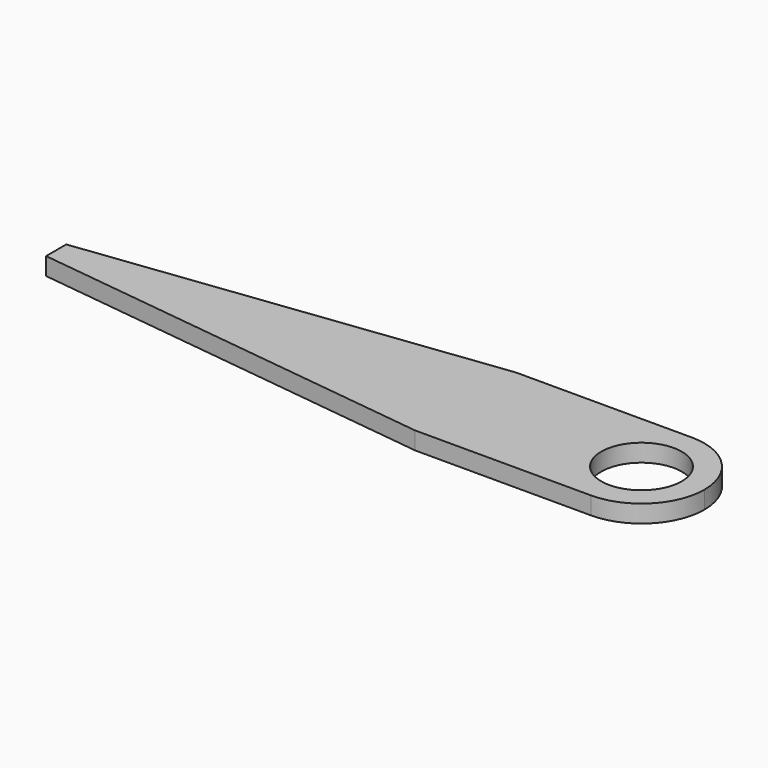
from build123d import *

# Parameters (mm, degrees)
F0_R     = 8
F1_DEPTH = 3.5


# Not quite as in the source:
# - the program builds the solid bodies; features that only make, move or delete a surface that nothing else refers to are left out


with BuildPart() as f1:
    # F0 (on Top) → F1 (new body)
    with BuildSketch(Plane.XY):
        with BuildLine():
            ThreePointArc((0, -12.5), (-12.5, 0), (0, 12.5))
            Line((0, 12.5), (-35, 12.5))
            Line((-35, 12.5), (-116.3887844346, 2.5067138408))
            Line((-116.3887844346, 2.5067138408), (-116.3887844346, -2.5067138408))
            Line((-116.3887844346, -2.5067138408), (-35, -12.5))
            Line((-35, -12.5), (0, -12.5))
        make_face()
        with BuildLine():
            ThreePointArc((0, -12.5), (8.8388347648, -8.8388347648), (12.5, 0))
            ThreePointArc((12.5, 0), (8.8388347648, 8.8388347648), (0, 12.5))
            ThreePointArc((0, 12.5), (-12.5, 0), (0, -12.5))
        make_face()
        Circle(F0_R, mode=Mode.SUBTRACT)
    extrude(amount=F1_DEPTH)


solid = f1.part
